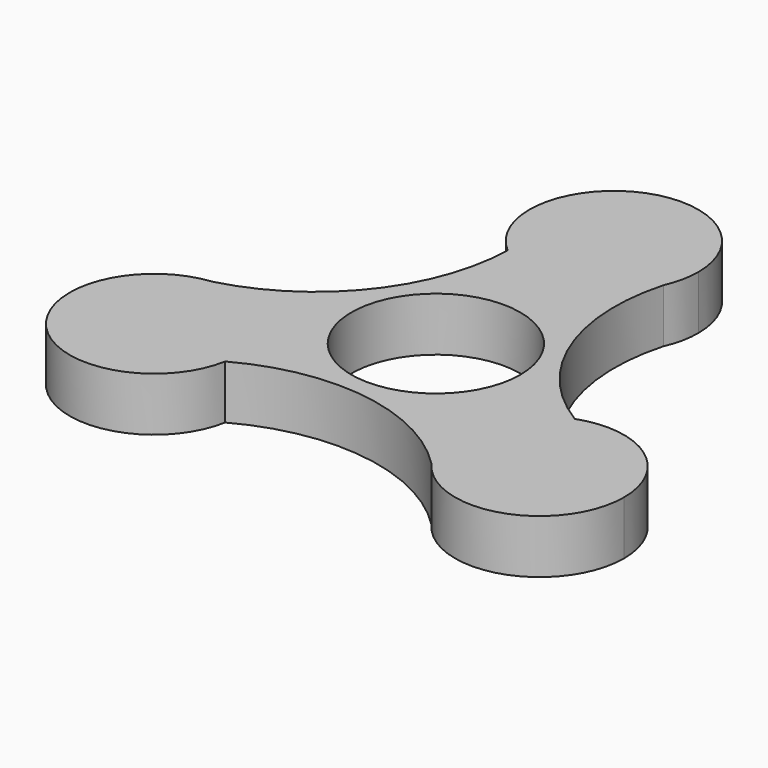
from build123d import *

# Parameters (mm, degrees)
F0_R     = 11
F1_DEPTH = 7


# Not quite as in the source:
# - a feature of the source that left no trace in its solid (it failed there, or was rolled back) is left out


with BuildPart() as f1:
    # F0 (on Top) → F1 (new body)
    with BuildSketch(Plane.XY):
        with BuildLine():
            ThreePointArc((10.0491768514, 24.5005127008), (2.4404784534, 18.2483589799), (-7.1242678109, 20.5930010332))
            ThreePointArc((-7.1242678109, 20.5930010332), (-12.6262898219, 5.3096518199), (-26.2426548303, -3.54741391))
            ThreePointArc((-26.2426548303, -3.54741391), (-17.732134245, -6.3123707797), (-14.0924093757, -14.4871093077))
            ThreePointArc((-14.0924093757, -14.4871093077), (-14.1373809935, -15.4807657603), (-14.2719281295, -16.4662974242))
            ThreePointArc((-14.2719281295, -16.4662974242), (1.7148515496, -13.5895136513), (16.1934779789, -20.9530987908))
            ThreePointArc((16.1934779789, -20.9530987908), (14.5833032273, -11.237695828), (21.3961959404, -4.126703609))
            ThreePointArc((21.3961959404, -4.126703609), (10.9114382722, 8.2798618313), (10.0491768514, 24.5005127008))
        make_face()
        Circle(F0_R, mode=Mode.SUBTRACT)
        with BuildLine():
            ThreePointArc((10.0491768514, 24.5005127008), (10.7596687999, 26.6874026373), (11, 28.9742186153))
            ThreePointArc((11, 28.9742186153), (-4.6169824604, 38.9583797198), (-7.1242678109, 20.5930010332))
            ThreePointArc((-7.1242678109, 20.5930010332), (2.4404784534, 18.2483589799), (10.0491768514, 24.5005127008))
        make_face()
        with BuildLine():
            ThreePointArc((-14.0924093757, -14.4871093077), (-17.732134245, -6.3123707797), (-26.2426548303, -3.54741391))
            ThreePointArc((-26.2426548303, -3.54741391), (-33.1610370706, -21.9635554634), (-14.2719281295, -16.4662974242))
            ThreePointArc((-14.2719281295, -16.4662974242), (-14.1373809935, -15.4807657603), (-14.0924093757, -14.4871093077))
        make_face()
        with BuildLine():
            ThreePointArc((36.0924093757, -14.4871093077), (31.4304552974, -5.4966046559), (21.3961959404, -4.126703609))
            ThreePointArc((21.3961959404, -4.126703609), (14.5833032273, -11.237695828), (16.1934779789, -20.9530987908))
            ThreePointArc((16.1934779789, -20.9530987908), (28.4918030448, -24.9486638137), (36.0924093757, -14.4871093077))
        make_face()
    extrude(amount=F1_DEPTH)


solid = f1.part
